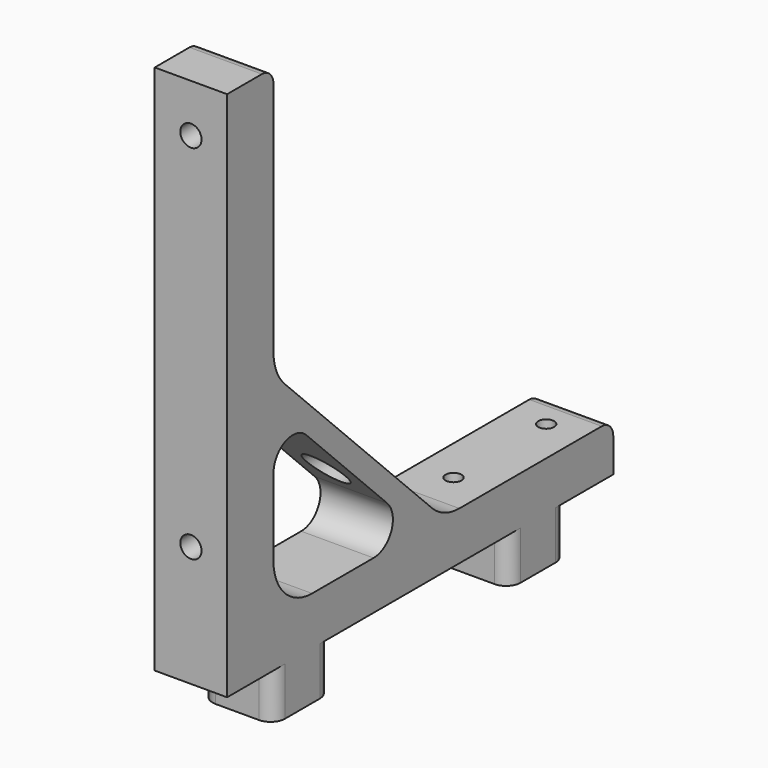
from build123d import *

# Parameters (mm, degrees)
F1_DEPTH  = 15
F2_DEPTH  = 15
F3_R      = 10
F4_R      = 5
F5_R      = 3
F7_D      = 4.4
F8_R      = 4
F9_DEPTH  = 23.5
F10_W     = 15
F10_H     = 15
F11_DEPTH = 10
F12_DEPTH = 10
F10_R     = 1.65
F13_DEPTH = 15
F14_R     = 3


with BuildPart() as f1:
    # F0 (on Right) → F1 (new body)
    with BuildSketch(Plane.YZ):
        with BuildLine():
            Line((-50, 0), (0, 0))
            Line((0, 0), (50, 0))
            Line((50, 0), (50, 10))
            Line((50, 10), (6, 10))
            Line((6, 10), (0, 10))
            Line((0, 10), (-28, 10))
            ThreePointArc((-28, 10), (-35.0710678119, 12.9289321881), (-38, 20))
            Line((-38, 20), (-38, 48))
            Line((-38, 48), (-38, 54))
            Line((-38, 54), (-38, 110))
            Line((-38, 110), (-50, 110))
            Line((-50, 110), (-50, 10))
            Line((-50, 10), (-50, 0))
        make_face()
    extrude(amount=F1_DEPTH)

    # F0 (on Right) → F2 (join, through all)
    with BuildSketch(Plane.YZ):
        Polygon((0, 10), (6, 10), (-38, 54), (-38, 48), align=None)
    extrude(amount=F2_DEPTH)

    # F3
    f3_edges = [f1.edges().sort_by_distance(p)[0] for p in [
        (7.5, 6, 10),
        (7.5, -38, 54),
    ]]
    fillet(f3_edges, radius=F3_R)

    # F4
    f4_edges = [f1.edges().sort_by_distance(p)[0] for p in [
        (7.5, 0, 10),
        (7.5, -38, 48),
    ]]
    fillet(f4_edges, radius=F4_R)

    # F5
    f5_edges = [f1.edges().sort_by_distance(p)[0] for p in [
        (7.5, 50, 10),
        (7.5, -38, 110),
    ]]
    fillet(f5_edges, radius=F5_R)

    # F7 (through all)
    with Locations(Plane.XZ.offset(50)):
        with Locations((7.5, 100), (7.5, 25)):
            Hole(F7_D / 2)

    # F8 (on Front) → F9 (cut)
    with BuildSketch(Plane.XZ):
        with Locations((7.5, 25)):
            Circle(F8_R)
    extrude(amount=F9_DEPTH, mode=Mode.SUBTRACT)

    # F10 (on face) → F11 (join)
    with BuildSketch(Plane(origin=(0, 0, 0), x_dir=(1, 0, 0), z_dir=(0, 0, -1))):
        with Locations((7.5, 30.5)):
            Rectangle(F10_W, F10_H)
    extrude(amount=F11_DEPTH)

    # F10 (on face) → F12 (join)
    with BuildSketch(Plane(origin=(0, 0, 0), x_dir=(1, 0, 0), z_dir=(0, 0, -1))):
        with Locations((7.5, -30.5)):
            Rectangle(F10_W, F10_H)
    extrude(amount=F12_DEPTH)

    # F10 (on face) → F13 (cut)
    with BuildSketch(Plane(origin=(0, 0, 0), x_dir=(1, 0, 0), z_dir=(0, 0, -1))):
        with Locations((7.5, -42)):
            Circle(F10_R)
        with Locations((7.5, -18)):
            Circle(F10_R)
        with Locations((7.5, 44)):
            Circle(F10_R)
    extrude(amount=-F13_DEPTH, mode=Mode.SUBTRACT)

    # F14
    f14_edges = [f1.edges().sort_by_distance(p)[0] for p in [
        (15, -38, -5),
        (0, -38, -5),
        (0, -23, -5),
        (15, 23, -5),
        (15, 38, -5),
        (0, 38, -5),
        (0, 23, -5),
        (15, -23, -5),
    ]]
    fillet(f14_edges, radius=F14_R)


solid = f1.part
